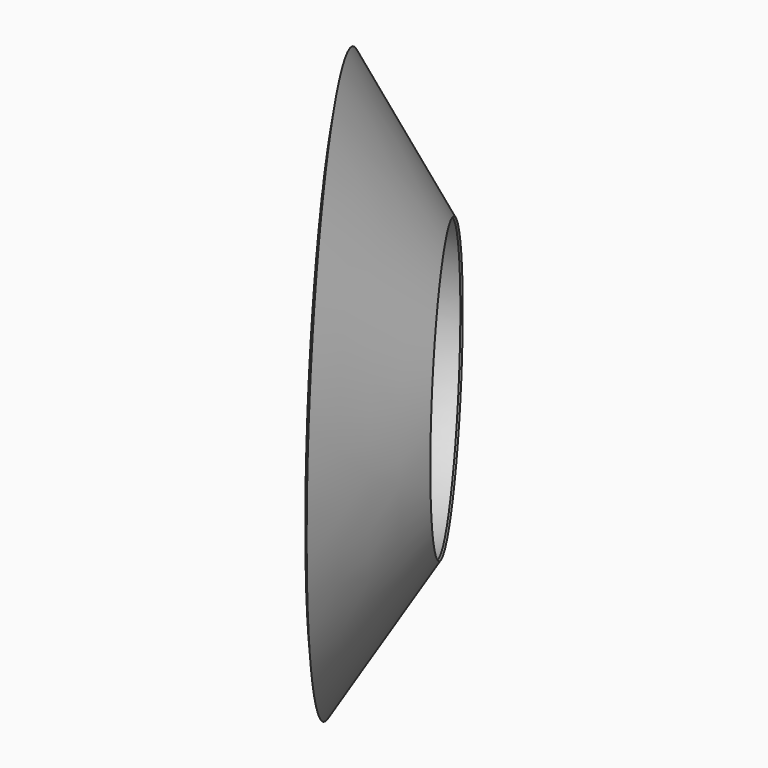
from build123d import *


with BuildPart() as f1:
    # F0 (on Top) → F1 (revolve)
    with BuildSketch(Plane.XY):
        with BuildLine():
            add(Edge.make_bspline(
                [(32.8465292277, -49.2566897612), (1.4788567079, -16.758781622), (29.3841917522, -12.91295474), (20.4192424175, 15.812341124), (6.9211326633, 24.0947962118), (31.4413485281, 53.533737281)],
                knots=[0.0158389184, 0.0158389184, 0.0158389184, 0.0158389184, 0.3912335435, 0.6229320327, 0.9972490619, 0.9972490619, 0.9972490619, 0.9972490619], degree=3))
            Line((32.8465292277, -49.2566897612), (32.8465292277, 53.533737281))
            Line((32.8465292277, 53.533737281), (31.4413485281, 53.533737281))
        make_face()
    revolve(axis=Axis((-30.8695323067, 119.0810969722, 0), (0.8359932827, 0.5487396754, 0)))


solid = f1.part
